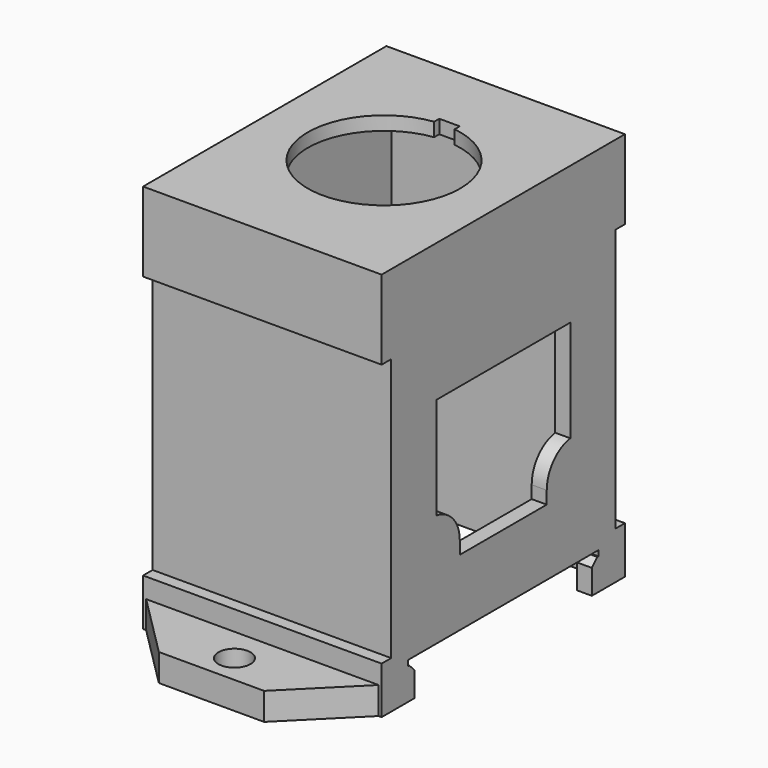
from build123d import *

# Parameters (mm, degrees)
F0_W         = 34.9
F0_H         = 44.5
F1_DEPTH     = 57
F2_W         = 30.5
F2_H         = 40.8
F3_DEPTH     = 55
F5_DEPTH     = 57.001
F6_W         = 1.75
F6_H         = 38.5
F7_DEPTH     = 34.901
F8_W         = 15.9
F8_H         = 6.8
F8_W_2       = 32.4
F8_H_2       = 4.6
F9_DEPTH     = 34.901
F10_W        = 34
F10_H        = 4
F11_DEPTH    = 9.3
F12_W        = 34
F12_H        = 4
F13_DEPTH    = 9.3
F14_SIZE     = 9.29999
F15_SIZE     = 1
F16_R        = 2.35
F17_DEPTH    = 4.001
F18_T1_DEPTH = 26.953787589
F18_T3_DEPTH = 26.953787589


# Not quite as in the source:
# - a fillet or chamfer that OpenCascade refuses, or shapes differently, is made with other operations: its cross-section is extruded or revolved along the edge and cut away or added
# - a fillet or chamfer is up to 0.001 mm smaller than in the source, because OpenCascade refuses the exact size


with BuildPart() as f1:
    # F0 (on Top) → F1 (new body)
    with BuildSketch(Plane.XY):
        with Locations((17.45, 22.6589083523)):
            Rectangle(F0_W, F0_H)
    extrude(amount=F1_DEPTH)

    # F2 (on face) → F3 (cut)
    with BuildSketch(Plane(origin=(0, 0, 0), x_dir=(1, 0, 0), z_dir=(0, 0, -1))):
        with Locations((17.45, -22.6589083523)):
            Rectangle(F2_W, F2_H)
    extrude(amount=-F3_DEPTH, mode=Mode.SUBTRACT)

    # F4 (on face) → F5 (cut, through all)
    with BuildSketch(Plane.XY.offset(57)):
        with BuildLine():
            Line((18.95, 33.2867875695), (18.95, 33.7075508028))
            ThreePointArc((18.95, 33.7075508028), (17.45, 33.8089083523), (15.95, 33.7075508028))
            Line((15.95, 33.7075508028), (15.95, 33.2867875695))
            Line((15.95, 33.2867875695), (18.95, 33.2867875695))
        make_face()
        with BuildLine():
            ThreePointArc((15.95, 33.7075508028), (10.1152368818, 14.2610663676), (28.6, 22.6589083523))
            ThreePointArc((28.6, 22.6589083523), (25.8478419847, 29.9936714704), (18.95, 33.7075508028))
            Line((18.95, 33.7075508028), (18.95, 33.2867875695))
            Line((18.95, 33.2867875695), (15.95, 33.2867875695))
            Line((15.95, 33.2867875695), (15.95, 33.7075508028))
        make_face()
        with BuildLine():
            ThreePointArc((15.95, 33.7075508028), (17.45, 33.8089083523), (18.95, 33.7075508028))
            Line((18.95, 33.7075508028), (18.95, 34.6477875695))
            Line((18.95, 34.6477875695), (15.95, 34.6477875695))
            Line((15.95, 34.6477875695), (15.95, 33.7075508028))
        make_face()
    extrude(amount=-F5_DEPTH, mode=Mode.SUBTRACT)

    # F6 (on face) → F7 (cut, through all)
    with BuildSketch(Plane(origin=(0, 0, 0), x_dir=(0, -1, 0), z_dir=(-1, 0, 0))):
        with Locations((-44.0339083523, 26.15)):
            Rectangle(F6_W, F6_H)
        with Locations((-1.2839083523, 26.15)):
            Rectangle(F6_W, F6_H)
    extrude(amount=-F7_DEPTH, mode=Mode.SUBTRACT)

    # F8 (on face) → F9 (cut, through all)
    with BuildSketch(Plane(origin=(0, 0, 0), x_dir=(0, -1, 0), z_dir=(-1, 0, 0))):
        Polygon((-10.4089083523, 36.8), (-34.9089083523, 36.8), (-34.9089083523, 21.9), (-30.6089083523, 21.9), (-14.7089083523, 21.9), (-10.4089083523, 21.9), align=None)
        with Locations((-22.6589083523, 18.5)):
            Rectangle(F8_W, F8_H)
        with Locations((-22.6589083523, 2.3)):
            Rectangle(F8_W_2, F8_H_2)
        Polygon((-40.0589083523, 4.6), (-38.8589083523, 4.6), (-6.4589083523, 4.6), (-5.2589083523, 4.6), (-5.2589083523, 5.4), (-40.0589083523, 5.4), align=None)
    extrude(amount=-F9_DEPTH, mode=Mode.SUBTRACT)

    # F10 (on face) → F11 (join)
    with BuildSketch(Plane.XZ.offset(-0.4089083523)):
        with Locations((17.45, 2)):
            Rectangle(F10_W, F10_H)
    extrude(amount=F11_DEPTH)

    # F12 (on face) → F13 (join)
    with BuildSketch(Plane(origin=(0, 44.9089083523, 0), x_dir=(-1, 0, 0), z_dir=(0, 1, 0))):
        with Locations((-17.45, 2)):
            Rectangle(F12_W, F12_H)
    extrude(amount=F13_DEPTH)

    # F14 (size 9.3 in the source; OpenCascade refuses exactly that, so slightly less here)
    f14_edges = [f1.edges().sort_by_distance(p)[0] for p in [
        (34.45, 54.208908, 2),
        (0.45, 54.208908, 2),
        (34.45, -8.891092, 2),
        (0.45, -8.891092, 2),
    ]]
    chamfer(f14_edges, length=F14_SIZE)

    # F15
    f15_edges = [f1.edges().sort_by_distance(p)[0] for p in [
        (1.1, 38.858908, 4.6),
        (1.1, 6.458908, 4.6),
        (33.8, 6.458908, 4.6),
        (33.8, 38.858908, 4.6),
    ]]
    chamfer(f15_edges, length=F15_SIZE)

    # F16 (on face) → F17 (cut, through all)
    with BuildSketch(Plane.XY.offset(4)):
        with Locations((17.45, -4.6910916477)):
            Circle(F16_R)
        with Locations((17.45, 50.0089083523)):
            Circle(F16_R)
    extrude(amount=-F17_DEPTH, mode=Mode.SUBTRACT)

    # F18: fillet of radius 5 on 4 edges, made by hand

    # F18_s2 → F18_t1 (cut)
    with BuildSketch(Plane.YZ.offset(-12.3768937945)):
        with BuildLine():
            ThreePointArc((30.6089083523, 16.9492424822), (31.8339911346, 20.2279617444), (34.9089083523, 21.9))
            Line((34.9089083523, 21.9), (30.6089083523, 21.9))
            Line((30.6089083523, 21.9), (30.6089083523, 16.9492424822))
        make_face()
        with BuildLine():
            ThreePointArc((10.4089083523, 21.9), (13.4838255699, 20.2279617444), (14.7089083523, 16.9492424822))
            Line((14.7089083523, 16.9492424822), (14.7089083523, 21.9))
            Line((14.7089083523, 21.9), (10.4089083523, 21.9))
        make_face()
    extrude(amount=F18_T1_DEPTH, mode=Mode.SUBTRACT)

    # F18_s4 → F18_t3 (cut)
    with BuildSketch(Plane.YZ.offset(20.3231062055)):
        with BuildLine():
            ThreePointArc((14.7089083523, 16.9492424822), (13.4838255699, 20.2279617444), (10.4089083523, 21.9))
            Line((10.4089083523, 21.9), (14.7089083523, 21.9))
            Line((14.7089083523, 21.9), (14.7089083523, 16.9492424822))
        make_face()
        with BuildLine():
            ThreePointArc((34.9089083523, 21.9), (31.8339911346, 20.2279617444), (30.6089083523, 16.9492424822))
            Line((30.6089083523, 16.9492424822), (30.6089083523, 21.9))
            Line((30.6089083523, 21.9), (34.9089083523, 21.9))
        make_face()
    extrude(amount=F18_T3_DEPTH, mode=Mode.SUBTRACT)


solid = f1.part
